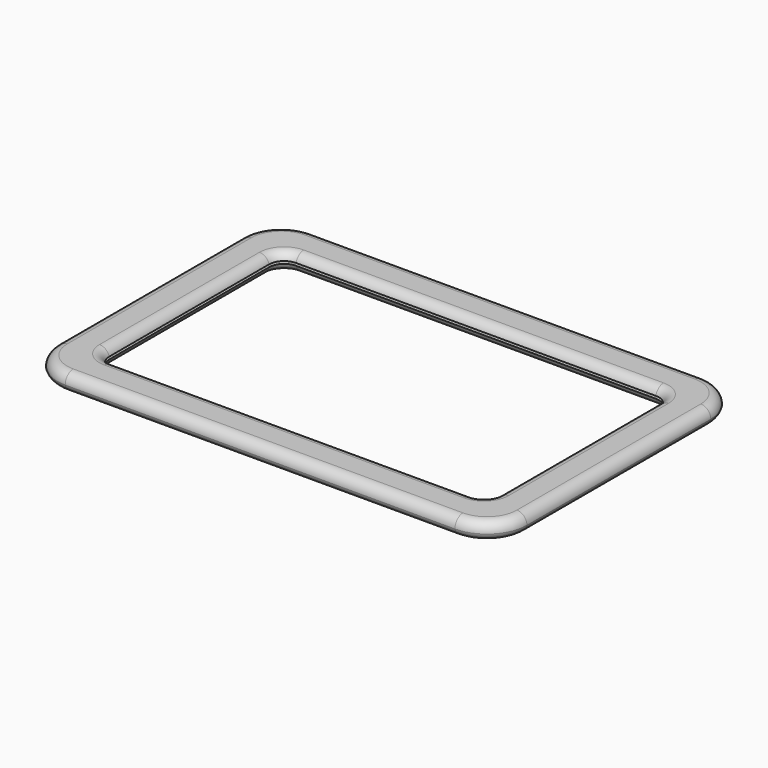
from build123d import *

# Parameters (mm, degrees)
F3_DEPTH     = 1.75
F4_DEPTH     = 12.5
F5_DEPTH     = 0.25
F8_T1_DEPTH  = 78
F8_T3_DEPTH  = 46
F8_T5_DEPTH  = 72
F8_T7_DEPTH  = 40
F8_T10_ANGLE = 90
F8_T12_ANGLE = 90
F8_T14_ANGLE = 90
F8_T16_ANGLE = 90
F8_T18_ANGLE = 90
F8_T20_ANGLE = 90
F8_T22_ANGLE = 90
F8_T24_ANGLE = 90
F9_T1_DEPTH  = 78
F9_T3_DEPTH  = 46
F9_T5_DEPTH  = 72
F9_T7_DEPTH  = 40
F9_T10_ANGLE = 90
F9_T12_ANGLE = 90
F9_T14_ANGLE = 90
F9_T16_ANGLE = 90
F9_T18_ANGLE = 90
F9_T20_ANGLE = 90
F9_T22_ANGLE = 90
F9_T24_ANGLE = 90


# Not quite as in the source:
# - a fillet or chamfer that OpenCascade refuses, or shapes differently, is made with other operations: its cross-section is extruded or revolved along the edge and cut away or added


with BuildPart() as f3:
    # F2 (on Top) → F3 (new body, symmetric)
    with BuildSketch(Plane.XY):
        with BuildLine():
            ThreePointArc((-47, -23), (-44.6568542495, -28.6568542495), (-39, -31))
            Line((-39, -31), (39, -31))
            ThreePointArc((39, -31), (44.6568542495, -28.6568542495), (47, -23))
            Line((47, -23), (47, 23))
            ThreePointArc((47, 23), (44.6568542495, 28.6568542495), (39, 31))
            Line((39, 31), (-39, 31))
            ThreePointArc((-39, 31), (-44.6568542495, 28.6568542495), (-47, 23))
            Line((-47, 23), (-47, -23))
        make_face()
    extrude(amount=F3_DEPTH, both=True)


with BuildPart() as f4:
    # F1 (on Top) → F4 (new body, symmetric)
    with BuildSketch(Plane.XY):
        with BuildLine():
            ThreePointArc((-39, -20), (-38.1213203436, -22.1213203436), (-36, -23))
            Line((-36, -23), (36, -23))
            ThreePointArc((36, -23), (38.1213203436, -22.1213203436), (39, -20))
            Line((39, -20), (39, 20))
            ThreePointArc((39, 20), (38.1213203436, 22.1213203436), (36, 23))
            Line((36, 23), (-36, 23))
            ThreePointArc((-36, 23), (-38.1213203436, 22.1213203436), (-39, 20))
            Line((-39, 20), (-39, -20))
        make_face()
    extrude(amount=F4_DEPTH, both=True)


with BuildPart() as f5:
    # F0 (on Top) → F5 (new body, symmetric)
    with BuildSketch(Plane.XY):
        with BuildLine():
            Line((40.5, 27), (-40.5, 27))
            ThreePointArc((-40.5, 27), (-42.267766953, 26.267766953), (-43, 24.5))
            Line((-43, 24.5), (-43, -24.5))
            ThreePointArc((-43, -24.5), (-42.267766953, -26.267766953), (-40.5, -27))
            Line((-40.5, -27), (40.5, -27))
            ThreePointArc((40.5, -27), (42.267766953, -26.267766953), (43, -24.5))
            Line((43, -24.5), (43, 24.5))
            ThreePointArc((43, 24.5), (42.267766953, 26.267766953), (40.5, 27))
        make_face()
    extrude(amount=F5_DEPTH, both=True)


with BuildPart() as f3_1:
    add(f3.part)

    # F6: cut F4
    add(f4.part, mode=Mode.SUBTRACT)

    # F7: cut F5
    add(f5.part, mode=Mode.SUBTRACT)

    # F8: fillet of radius 2 on 16 edges, made by hand

    # F8_s2 → F8_t1 (cut)
    with BuildSketch(Plane.YZ.offset(-39)):
        with BuildLine():
            ThreePointArc((29, 1.75), (30.4142135624, 1.1642135624), (31, -0.25))
            Line((31, -0.25), (31, 1.75))
            Line((31, 1.75), (29, 1.75))
        make_face()
        with BuildLine():
            ThreePointArc((-29, 1.75), (-30.4142135624, 1.1642135624), (-31, -0.25))
            Line((-31, -0.25), (-31, 1.75))
            Line((-31, 1.75), (-29, 1.75))
        make_face()
    extrude(amount=F8_T1_DEPTH, mode=Mode.SUBTRACT)

    # F8_s4 → F8_t3 (cut)
    with BuildSketch(Plane.XZ.offset(-23)):
        with BuildLine():
            ThreePointArc((-47, -0.25), (-46.4142135624, 1.1642135624), (-45, 1.75))
            Line((-45, 1.75), (-47, 1.75))
            Line((-47, 1.75), (-47, -0.25))
        make_face()
        with BuildLine():
            ThreePointArc((45, 1.75), (46.4142135624, 1.1642135624), (47, -0.25))
            Line((47, -0.25), (47, 1.75))
            Line((47, 1.75), (45, 1.75))
        make_face()
    extrude(amount=F8_T3_DEPTH, mode=Mode.SUBTRACT)

    # F8_s6 → F8_t5 (cut)
    with BuildSketch(Plane.YZ.offset(-36)):
        with BuildLine():
            ThreePointArc((-24.9364916731, 1.75), (-23.7117468017, 1.3311388301), (-23, 0.25))
            Line((-23, 0.25), (-23, 1.75))
            Line((-23, 1.75), (-24.9364916731, 1.75))
        make_face()
        with BuildLine():
            ThreePointArc((24.9364916731, 1.75), (23.7117468017, 1.3311388301), (23, 0.25))
            Line((23, 0.25), (23, 1.75))
            Line((23, 1.75), (24.9364916731, 1.75))
        make_face()
    extrude(amount=F8_T5_DEPTH, mode=Mode.SUBTRACT)

    # F8_s8 → F8_t7 (cut)
    with BuildSketch(Plane.XZ.offset(-20)):
        with BuildLine():
            ThreePointArc((40.9364916731, 1.75), (39.7117468017, 1.3311388301), (39, 0.25))
            Line((39, 0.25), (39, 1.75))
            Line((39, 1.75), (40.9364916731, 1.75))
        make_face()
        with BuildLine():
            ThreePointArc((-40.9364916731, 1.75), (-39.7117468017, 1.3311388301), (-39, 0.25))
            Line((-39, 0.25), (-39, 1.75))
            Line((-39, 1.75), (-40.9364916731, 1.75))
        make_face()
    extrude(amount=F8_T7_DEPTH, mode=Mode.SUBTRACT)

    # F8_s9 → F8_t10 (revolve, cut)
    with BuildSketch(Plane.YZ.offset(-39)):
        with BuildLine():
            ThreePointArc((31, -0.25), (30.4142135624, 1.1642135624), (29, 1.75))
            Line((29, 1.75), (31, 1.75))
            Line((31, 1.75), (31, -0.25))
        make_face()
    revolve(axis=Axis((-39, 23, 1.75), (0, 0, 1)), revolution_arc=F8_T10_ANGLE, mode=Mode.SUBTRACT)

    # F8_s11 → F8_t12 (revolve, cut)
    with BuildSketch(Plane.XZ.offset(-23)):
        with BuildLine():
            ThreePointArc((45, 1.75), (46.4142135624, 1.1642135624), (47, -0.25))
            Line((47, -0.25), (47, 1.75))
            Line((47, 1.75), (45, 1.75))
        make_face()
    revolve(axis=Axis((39, 23, 1.75), (0, 0, 1)), revolution_arc=F8_T12_ANGLE, mode=Mode.SUBTRACT)

    # F8_s13 → F8_t14 (revolve, cut)
    with BuildSketch(Plane.XZ.offset(23)):
        with BuildLine():
            ThreePointArc((-45, 1.75), (-46.4142135624, 1.1642135624), (-47, -0.25))
            Line((-47, -0.25), (-47, 1.75))
            Line((-47, 1.75), (-45, 1.75))
        make_face()
    revolve(axis=Axis((-39, -23, 1.75), (0, 0, 1)), revolution_arc=F8_T14_ANGLE, mode=Mode.SUBTRACT)

    # F8_s15 → F8_t16 (revolve, cut)
    with BuildSketch(Plane.YZ.offset(39)):
        with BuildLine():
            ThreePointArc((-29, 1.75), (-30.4142135624, 1.1642135624), (-31, -0.25))
            Line((-31, -0.25), (-31, 1.75))
            Line((-31, 1.75), (-29, 1.75))
        make_face()
    revolve(axis=Axis((39, -23, 1.75), (0, 0, 1)), revolution_arc=F8_T16_ANGLE, mode=Mode.SUBTRACT)

    # F8_s17 → F8_t18 (revolve, cut)
    with BuildSketch(Plane.XZ.offset(20)):
        with BuildLine():
            ThreePointArc((-40.9364916731, 1.75), (-39.7117468017, 1.3311388301), (-39, 0.25))
            Line((-39, 0.25), (-39, 1.75))
            Line((-39, 1.75), (-40.9364916731, 1.75))
        make_face()
    revolve(axis=Axis((-36, -20, 1.75), (0, 0, 1)), revolution_arc=F8_T18_ANGLE, mode=Mode.SUBTRACT)

    # F8_s19 → F8_t20 (revolve, cut)
    with BuildSketch(Plane.YZ.offset(36)):
        with BuildLine():
            ThreePointArc((-24.9364916731, 1.75), (-23.7117468017, 1.3311388301), (-23, 0.25))
            Line((-23, 0.25), (-23, 1.75))
            Line((-23, 1.75), (-24.9364916731, 1.75))
        make_face()
    revolve(axis=Axis((36, -20, 1.75), (0, 0, 1)), revolution_arc=F8_T20_ANGLE, mode=Mode.SUBTRACT)

    # F8_s21 → F8_t22 (revolve, cut)
    with BuildSketch(Plane.XZ.offset(-20)):
        with BuildLine():
            ThreePointArc((40.9364916731, 1.75), (39.7117468017, 1.3311388301), (39, 0.25))
            Line((39, 0.25), (39, 1.75))
            Line((39, 1.75), (40.9364916731, 1.75))
        make_face()
    revolve(axis=Axis((36, 20, 1.75), (0, 0, 1)), revolution_arc=F8_T22_ANGLE, mode=Mode.SUBTRACT)

    # F8_s23 → F8_t24 (revolve, cut)
    with BuildSketch(Plane.YZ.offset(-36)):
        with BuildLine():
            ThreePointArc((24.9364916731, 1.75), (23.7117468017, 1.3311388301), (23, 0.25))
            Line((23, 0.25), (23, 1.75))
            Line((23, 1.75), (24.9364916731, 1.75))
        make_face()
    revolve(axis=Axis((-36, 20, 1.75), (0, 0, 1)), revolution_arc=F8_T24_ANGLE, mode=Mode.SUBTRACT)

    # F9: fillet of radius 2 on 16 edges, made by hand

    # F9_s2 → F9_t1 (cut)
    with BuildSketch(Plane.YZ.offset(-39)):
        with BuildLine():
            ThreePointArc((31, -0.25), (30.2882531983, -1.3311388301), (29.0635083269, -1.75))
            Line((29.0635083269, -1.75), (29.0635083269, -1.79))
            Line((29.0635083269, -1.79), (31, -1.79))
            Line((31, -1.79), (31.04, -1.75))
            ThreePointArc((31.04, -1.75), (31.04, -1), (31.0387298335, -0.26))
            Line((31.0387298335, -0.26), (31, -0.25))
        make_face()
        with BuildLine():
            ThreePointArc((-29.0635083269, -1.75), (-30.2882531983, -1.3311388301), (-31, -0.25))
            Line((-31, -0.25), (-31.0387298335, -0.26))
            ThreePointArc((-31.0387298335, -0.26), (-31.04, -1), (-31.04, -1.75))
            Line((-31.04, -1.75), (-31, -1.79))
            Line((-31, -1.79), (-29.0635083269, -1.79))
            Line((-29.0635083269, -1.79), (-29.0635083269, -1.75))
        make_face()
    extrude(amount=F9_T1_DEPTH, mode=Mode.SUBTRACT)

    # F9_s4 → F9_t3 (cut)
    with BuildSketch(Plane.XZ.offset(-23)):
        with BuildLine():
            ThreePointArc((-47, -0.25), (-46.2882531983, -1.3311388301), (-45.0635083269, -1.75))
            Line((-45.0635083269, -1.75), (-45.0635083269, -1.79))
            Line((-45.0635083269, -1.79), (-47, -1.79))
            Line((-47, -1.79), (-47.04, -1.75))
            ThreePointArc((-47.04, -1.75), (-47.04, -1), (-47.0387298335, -0.26))
            Line((-47.0387298335, -0.26), (-47, -0.25))
        make_face()
        with BuildLine():
            ThreePointArc((45.0635083269, -1.75), (46.2882531983, -1.3311388301), (47, -0.25))
            Line((47, -0.25), (47.0387298335, -0.26))
            ThreePointArc((47.0387298335, -0.26), (47.04, -1), (47.04, -1.75))
            Line((47.04, -1.75), (47, -1.79))
            Line((47, -1.79), (45.0635083269, -1.79))
            Line((45.0635083269, -1.79), (45.0635083269, -1.75))
        make_face()
    extrude(amount=F9_T3_DEPTH, mode=Mode.SUBTRACT)

    # F9_s6 → F9_t5 (cut)
    with BuildSketch(Plane.YZ.offset(-36)):
        with BuildLine():
            ThreePointArc((-24.9364916731, -1.75), (-23.7117468017, -1.3311388301), (-23, -0.25))
            Line((-23, -0.25), (-22.9612701665, -0.26))
            ThreePointArc((-22.9612701665, -0.26), (-22.96, -1), (-22.96, -1.75))
            Line((-22.96, -1.75), (-23, -1.79))
            Line((-23, -1.79), (-24.9364916731, -1.79))
            Line((-24.9364916731, -1.79), (-24.9364916731, -1.75))
        make_face()
        with BuildLine():
            ThreePointArc((24.9364916731, -1.75), (23.7117468017, -1.3311388301), (23, -0.25))
            Line((23, -0.25), (22.9612701665, -0.26))
            ThreePointArc((22.9612701665, -0.26), (22.96, -1), (22.96, -1.75))
            Line((22.96, -1.75), (23, -1.79))
            Line((23, -1.79), (24.9364916731, -1.79))
            Line((24.9364916731, -1.79), (24.9364916731, -1.75))
        make_face()
    extrude(amount=F9_T5_DEPTH, mode=Mode.SUBTRACT)

    # F9_s8 → F9_t7 (cut)
    with BuildSketch(Plane.XZ.offset(-20)):
        with BuildLine():
            ThreePointArc((40.9364916731, -1.75), (39.7117468017, -1.3311388301), (39, -0.25))
            Line((39, -0.25), (38.9612701665, -0.26))
            ThreePointArc((38.9612701665, -0.26), (38.96, -1), (38.96, -1.75))
            Line((38.96, -1.75), (39, -1.79))
            Line((39, -1.79), (40.9364916731, -1.79))
            Line((40.9364916731, -1.79), (40.9364916731, -1.75))
        make_face()
        with BuildLine():
            ThreePointArc((-40.9364916731, -1.75), (-39.7117468017, -1.3311388301), (-39, -0.25))
            Line((-39, -0.25), (-38.9612701665, -0.26))
            ThreePointArc((-38.9612701665, -0.26), (-38.96, -1), (-38.96, -1.75))
            Line((-38.96, -1.75), (-39, -1.79))
            Line((-39, -1.79), (-40.9364916731, -1.79))
            Line((-40.9364916731, -1.79), (-40.9364916731, -1.75))
        make_face()
    extrude(amount=F9_T7_DEPTH, mode=Mode.SUBTRACT)

    # F9_s9 → F9_t10 (revolve, cut)
    with BuildSketch(Plane.YZ.offset(-39)):
        with BuildLine():
            ThreePointArc((31, -0.25), (30.2882531983, -1.3311388301), (29.0635083269, -1.75))
            Line((29.0635083269, -1.75), (29.0635083269, -1.79))
            Line((29.0635083269, -1.79), (31, -1.79))
            Line((31, -1.79), (31.04, -1.75))
            ThreePointArc((31.04, -1.75), (31.04, -1), (31.0387298335, -0.26))
            Line((31.0387298335, -0.26), (31, -0.25))
        make_face()
    revolve(axis=Axis((-39, 23, -1.75), (0, 0, 1)), revolution_arc=F9_T10_ANGLE, mode=Mode.SUBTRACT)

    # F9_s11 → F9_t12 (revolve, cut)
    with BuildSketch(Plane.XZ.offset(-23)):
        with BuildLine():
            ThreePointArc((45.0635083269, -1.75), (46.2882531983, -1.3311388301), (47, -0.25))
            Line((47, -0.25), (47.0387298335, -0.26))
            ThreePointArc((47.0387298335, -0.26), (47.04, -1), (47.04, -1.75))
            Line((47.04, -1.75), (47, -1.79))
            Line((47, -1.79), (45.0635083269, -1.79))
            Line((45.0635083269, -1.79), (45.0635083269, -1.75))
        make_face()
    revolve(axis=Axis((39, 23, -1.75), (0, 0, 1)), revolution_arc=F9_T12_ANGLE, mode=Mode.SUBTRACT)

    # F9_s13 → F9_t14 (revolve, cut)
    with BuildSketch(Plane.XZ.offset(23)):
        with BuildLine():
            ThreePointArc((-45.0635083269, -1.75), (-46.2882531983, -1.3311388301), (-47, -0.25))
            Line((-47, -0.25), (-47.0387298335, -0.26))
            ThreePointArc((-47.0387298335, -0.26), (-47.04, -1), (-47.04, -1.75))
            Line((-47.04, -1.75), (-47, -1.79))
            Line((-47, -1.79), (-45.0635083269, -1.79))
            Line((-45.0635083269, -1.79), (-45.0635083269, -1.75))
        make_face()
    revolve(axis=Axis((-39, -23, -1.75), (0, 0, 1)), revolution_arc=F9_T14_ANGLE, mode=Mode.SUBTRACT)

    # F9_s15 → F9_t16 (revolve, cut)
    with BuildSketch(Plane.YZ.offset(39)):
        with BuildLine():
            ThreePointArc((-29.0635083269, -1.75), (-30.2882531983, -1.3311388301), (-31, -0.25))
            Line((-31, -0.25), (-31.0387298335, -0.26))
            ThreePointArc((-31.0387298335, -0.26), (-31.04, -1), (-31.04, -1.75))
            Line((-31.04, -1.75), (-31, -1.79))
            Line((-31, -1.79), (-29.0635083269, -1.79))
            Line((-29.0635083269, -1.79), (-29.0635083269, -1.75))
        make_face()
    revolve(axis=Axis((39, -23, -1.75), (0, 0, 1)), revolution_arc=F9_T16_ANGLE, mode=Mode.SUBTRACT)

    # F9_s17 → F9_t18 (revolve, cut)
    with BuildSketch(Plane.XZ.offset(20)):
        with BuildLine():
            ThreePointArc((-40.9364916731, -1.75), (-39.7117468017, -1.3311388301), (-39, -0.25))
            Line((-39, -0.25), (-38.9612701665, -0.26))
            ThreePointArc((-38.9612701665, -0.26), (-38.96, -1), (-38.96, -1.75))
            Line((-38.96, -1.75), (-39, -1.79))
            Line((-39, -1.79), (-40.9364916731, -1.79))
            Line((-40.9364916731, -1.79), (-40.9364916731, -1.75))
        make_face()
    revolve(axis=Axis((-36, -20, -1.75), (0, 0, 1)), revolution_arc=F9_T18_ANGLE, mode=Mode.SUBTRACT)

    # F9_s19 → F9_t20 (revolve, cut)
    with BuildSketch(Plane.YZ.offset(36)):
        with BuildLine():
            ThreePointArc((-24.9364916731, -1.75), (-23.7117468017, -1.3311388301), (-23, -0.25))
            Line((-23, -0.25), (-22.9612701665, -0.26))
            ThreePointArc((-22.9612701665, -0.26), (-22.96, -1), (-22.96, -1.75))
            Line((-22.96, -1.75), (-23, -1.79))
            Line((-23, -1.79), (-24.9364916731, -1.79))
            Line((-24.9364916731, -1.79), (-24.9364916731, -1.75))
        make_face()
    revolve(axis=Axis((36, -20, -1.75), (0, 0, 1)), revolution_arc=F9_T20_ANGLE, mode=Mode.SUBTRACT)

    # F9_s21 → F9_t22 (revolve, cut)
    with BuildSketch(Plane.XZ.offset(-20)):
        with BuildLine():
            ThreePointArc((40.9364916731, -1.75), (39.7117468017, -1.3311388301), (39, -0.25))
            Line((39, -0.25), (38.9612701665, -0.26))
            ThreePointArc((38.9612701665, -0.26), (38.96, -1), (38.96, -1.75))
            Line((38.96, -1.75), (39, -1.79))
            Line((39, -1.79), (40.9364916731, -1.79))
            Line((40.9364916731, -1.79), (40.9364916731, -1.75))
        make_face()
    revolve(axis=Axis((36, 20, -1.75), (0, 0, 1)), revolution_arc=F9_T22_ANGLE, mode=Mode.SUBTRACT)

    # F9_s23 → F9_t24 (revolve, cut)
    with BuildSketch(Plane.YZ.offset(-36)):
        with BuildLine():
            ThreePointArc((24.9364916731, -1.75), (23.7117468017, -1.3311388301), (23, -0.25))
            Line((23, -0.25), (22.9612701665, -0.26))
            ThreePointArc((22.9612701665, -0.26), (22.96, -1), (22.96, -1.75))
            Line((22.96, -1.75), (23, -1.79))
            Line((23, -1.79), (24.9364916731, -1.79))
            Line((24.9364916731, -1.79), (24.9364916731, -1.75))
        make_face()
    revolve(axis=Axis((-36, 20, -1.75), (0, 0, 1)), revolution_arc=F9_T24_ANGLE, mode=Mode.SUBTRACT)


solid = f3_1.part
